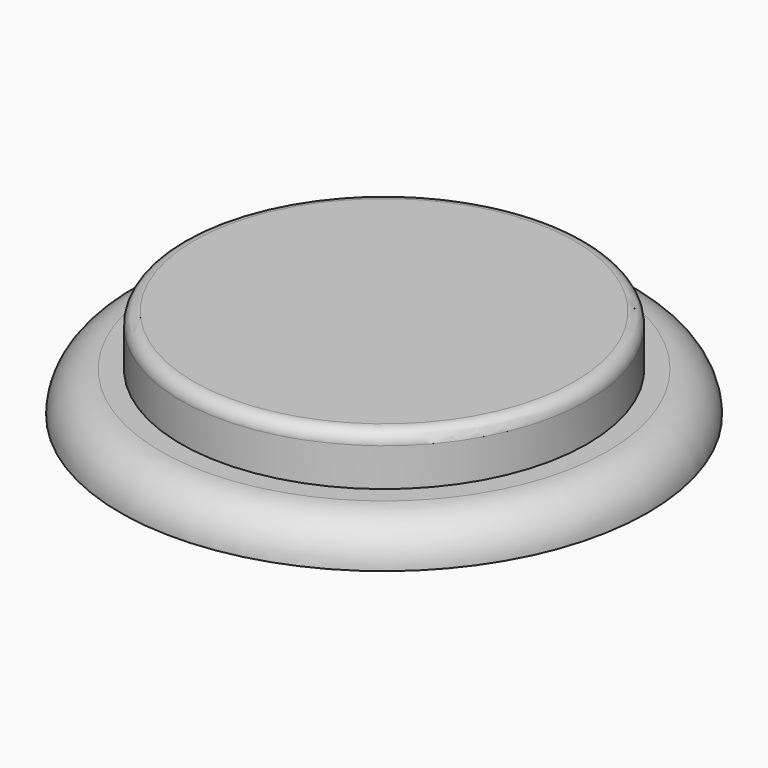
from build123d import *

# Parameters (mm, degrees)
F0_R     = 16.5
F1_DEPTH = 2.54
F2_R     = 12.7
F3_DEPTH = 3.175
F4_R     = 2.53999
F5_R     = 0.79375


# Not quite as in the source:
# - a fillet or chamfer is up to 0.001 mm smaller than in the source, because OpenCascade refuses the exact size


with BuildPart() as f1:
    # F0 (on Top) → F1 (new body)
    with BuildSketch(Plane.XY):
        Circle(F0_R)
    extrude(amount=F1_DEPTH)

    # F2 (on face) → F3 (join)
    with BuildSketch(Plane.XY.offset(2.54)):
        Circle(F2_R)
    extrude(amount=F3_DEPTH)

    # F4 (radius 2.54 in the source; OpenCascade refuses exactly that, so slightly less here)
    f4_edges = [f1.edges().sort_by_distance(p)[0] for p in [
        (-16.5, 0, 2.54),
    ]]
    fillet(f4_edges, radius=F4_R)

    # F5
    f5_edges = [f1.edges().sort_by_distance(p)[0] for p in [
        (-12.7, 0, 5.715),
    ]]
    fillet(f5_edges, radius=F5_R)


solid = f1.part
